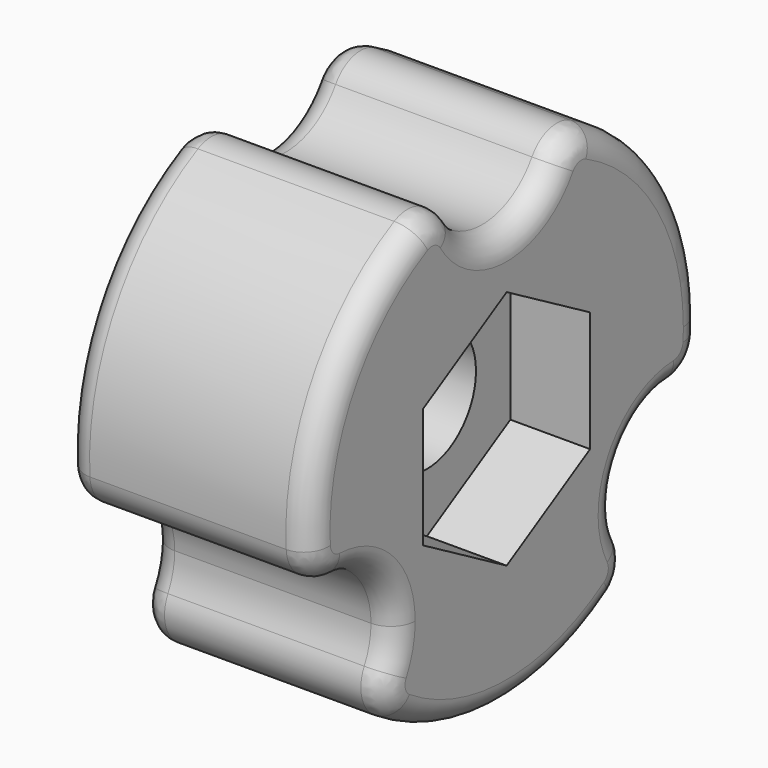
from build123d import *

# Parameters (mm, degrees)
F1_DEPTH = 20
F0_R     = 5
F2_DEPTH = 13.5
F3_R     = 3
F4_R     = 2


with BuildPart() as f1:
    # F0 (on Right) → F1 (new body)
    with BuildSketch(Plane.YZ):
        with BuildLine():
            ThreePointArc((19.5071432023, -4.4126368631), (19.8764039007, -2.2200378324), (20, 0))
            ThreePointArc((20, 0), (16.1034517977, 11.8608111105), (5.93211598, 19.1))
            ThreePointArc((5.93211598, 19.1), (0, 14), (-5.93211598, 19.1))
            ThreePointArc((-5.93211598, 19.1), (-17.3205080757, 10), (-19.5071432023, -4.4126368631))
            ThreePointArc((-19.5071432023, -4.4126368631), (-13.9381871831, -5.0442048691), (-11.3205080757, -10))
            ThreePointArc((-11.3205080757, -10), (-11.9134346935, -12.6006840331), (-13.5750272223, -14.6873631369))
            ThreePointArc((-13.5750272223, -14.6873631369), (0, -20), (13.5750272223, -14.6873631369))
            ThreePointArc((13.5750272223, -14.6873631369), (12.124355653, -7), (19.5071432023, -4.4126368631))
        make_face()
        Polygon((-8.4998142676, 4.9077989719), (0.0003714525, 9.8149545692), (8.5001857202, 4.9071555973), (8.4998142676, -4.9077989719), (-0.0003714525, -9.8149545692), (-8.5001857202, -4.9071555973), align=None, mode=Mode.SUBTRACT)
    extrude(amount=F1_DEPTH)

    # F0 (on Right) → F2 (join)
    with BuildSketch(Plane.YZ):
        Polygon((8.5001857202, 4.9071555973), (0.0003714525, 9.8149545692), (-8.4998142676, 4.9077989719), (-8.5001857202, -4.9071555973), (-0.0003714525, -9.8149545692), (8.4998142676, -4.9077989719), align=None)
        Circle(F0_R, mode=Mode.SUBTRACT)
    extrude(amount=F2_DEPTH)

    # F3
    f3_edges = [f1.edges().sort_by_distance(p)[0] for p in [
        (10, -19.507143, -4.412637),
        (10, -13.575027, -14.687363),
        (10, -5.932116, 19.1),
        (10, 5.932116, 19.1),
        (10, 19.507143, -4.412637),
        (10, 13.575027, -14.687363),
    ]]
    fillet(f3_edges, radius=F3_R)

    # F4
    f4_edges = [f1.edges().sort_by_distance(p)[0] for p in [
        (20, 0, -20),
        (0, 0, 14),
    ]]
    fillet(f4_edges, radius=F4_R)


solid = f1.part
